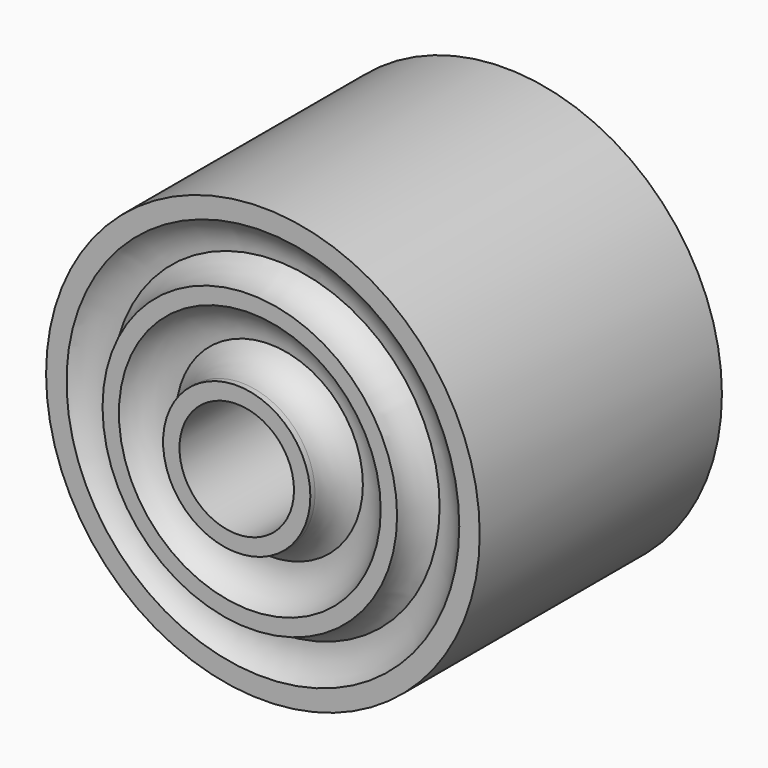
from build123d import *

# Parameters (mm, degrees)
F0_R      = 9
F0_R_2    = 7
F1_DEPTH  = 45
F3_R      = 16
F3_R_2    = 9
F4_DEPTH  = 35
F6_R      = 18
F6_R_2    = 16
F7_DEPTH  = 41
F9_R      = 26.5
F9_R_2    = 24
F10_DEPTH = 37
F12_R     = 24
F12_R_2   = 18
F13_DEPTH = 33


# Not quite as in the source:
# - a fillet or chamfer that OpenCascade refuses, or shapes differently, is made with other operations: its cross-section is extruded or revolved along the edge and cut away or added


with BuildPart() as f1:
    # F0 (on Front) → F1 (new body)
    with BuildSketch(Plane.XZ):
        Circle(F0_R)
        Circle(F0_R_2, mode=Mode.SUBTRACT)
    extrude(amount=F1_DEPTH)

    # F3 (on offset) → F4 (join)
    with BuildSketch(Plane.XZ.offset(5)):
        Circle(F3_R)
        Circle(F3_R_2, mode=Mode.SUBTRACT)
    extrude(amount=F4_DEPTH)

    # F6 (on offset) → F7 (join)
    with BuildSketch(Plane.XZ.offset(2)):
        Circle(F6_R)
        Circle(F6_R_2, mode=Mode.SUBTRACT)
    extrude(amount=F7_DEPTH)



with BuildPart() as f10:
    # F9 (on offset) → F10 (new body)
    with BuildSketch(Plane.XZ.offset(4)):
        Circle(F9_R)
        Circle(F9_R_2, mode=Mode.SUBTRACT)
    extrude(amount=F10_DEPTH)


with BuildPart() as f1_1:
    add(f1.part)

    add(f10.part)  # F13 merges F10
    # F12 (on offset) → F13 (join)
    with BuildSketch(Plane.XZ.offset(6)):
        Circle(F12_R)
        Circle(F12_R_2, mode=Mode.SUBTRACT)
    extrude(amount=F13_DEPTH)

    # F14: fillet of radius 5 on 2 edges, made by hand

    # F14_s1 → F14_t2 (revolve)
    with BuildSketch(Plane.XY):
        with BuildLine():
            ThreePointArc((16, -43), (14.1560370926, -40.8166998673), (11.417424305, -40))
            Line((11.417424305, -40), (16, -40))
            Line((16, -40), (16, -43))
        make_face()
    revolve(axis=Axis((0, -40, 0), (0, -1, 0)))

    # F14_s3 → F14_t4 (revolve)
    with BuildSketch(Plane.XY):
        with BuildLine():
            ThreePointArc((24, -41), (22.2360679775, -39.527864045), (20, -39))
            Line((20, -39), (24, -39))
            Line((24, -39), (24, -41))
        make_face()
    revolve(axis=Axis((0, -39, 0), (0, -1, 0)))

    # F15: fillet of radius 5 on 2 edges, made by hand

    # F15_s1 → F15_t2 (revolve)
    with BuildSketch(Plane.XY):
        with BuildLine():
            ThreePointArc((11.417424305, -40), (9.6461006859, -41.8230248202), (9, -44.2813902858))
            Line((9, -44.2813902858), (9, -40))
            Line((9, -40), (11.417424305, -40))
        make_face()
    revolve(axis=Axis((0, -40, 0), (0, -1, 0)))

    # F15_s3 → F15_t4 (revolve)
    with BuildSketch(Plane.XY):
        with BuildLine():
            ThreePointArc((20, -39), (18.527864045, -40.7639320225), (18, -43))
            Line((18, -43), (18, -39))
            Line((18, -39), (20, -39))
        make_face()
    revolve(axis=Axis((0, -39, 0), (0, -1, 0)))

    # F16: fillet of radius 5 on 2 edges, made by hand

    # F16_s1 → F16_t2 (revolve)
    with BuildSketch(Plane.XY):
        with BuildLine():
            ThreePointArc((16, -2), (14.1560370926, -4.1833001327), (11.417424305, -5))
            Line((11.417424305, -5), (16, -5))
            Line((16, -5), (16, -2))
        make_face()
    revolve(axis=Axis((0, -5, 0), (0, -1, 0)))

    # F16_s3 → F16_t4 (revolve)
    with BuildSketch(Plane.XY):
        with BuildLine():
            ThreePointArc((24, -4), (22.2360679775, -5.472135955), (20, -6))
            Line((20, -6), (24, -6))
            Line((24, -6), (24, -4))
        make_face()
    revolve(axis=Axis((0, -6, 0), (0, -1, 0)))

    # F17: fillet of radius 5 on 2 edges, made by hand

    # F17_s1 → F17_t2 (revolve)
    with BuildSketch(Plane.XY):
        with BuildLine():
            ThreePointArc((11.417424305, -5), (9.6461006859, -3.1769751798), (9, -0.7186097142))
            Line((9, -0.7186097142), (9, -5))
            Line((9, -5), (11.417424305, -5))
        make_face()
    revolve(axis=Axis((0, -5, 0), (0, -1, 0)))

    # F17_s3 → F17_t4 (revolve)
    with BuildSketch(Plane.XY):
        with BuildLine():
            ThreePointArc((20, -6), (18.527864045, -4.2360679775), (18, -2))
            Line((18, -2), (18, -6))
            Line((18, -6), (20, -6))
        make_face()
    revolve(axis=Axis((0, -6, 0), (0, -1, 0)))


solid = f1_1.part
